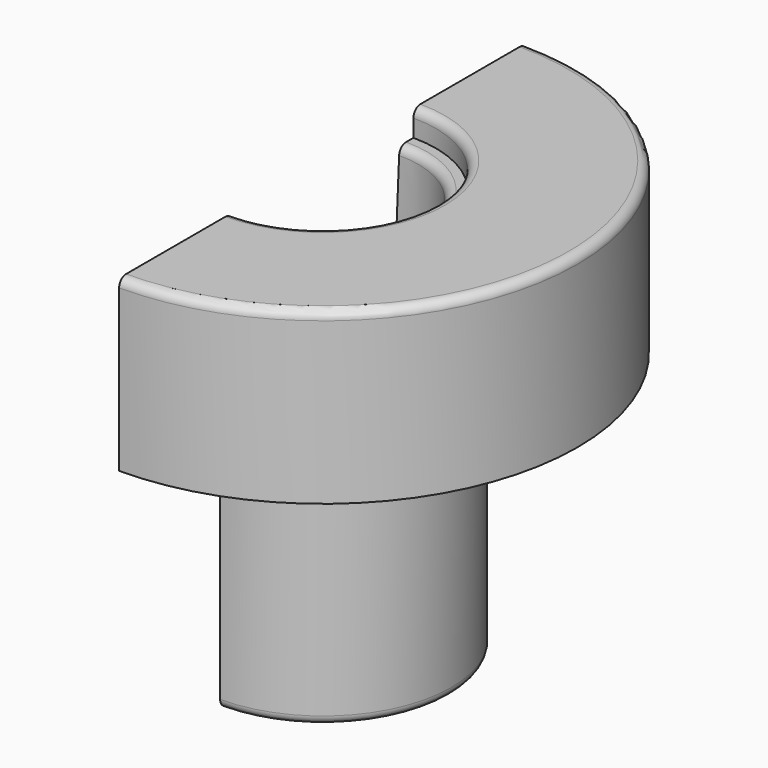
from build123d import *

# Parameters (mm, degrees)
F0_R         = 14.75
F1_DEPTH     = 30
F2_R         = 29.25
F3_DEPTH     = 19.5
F6_R         = 1
F8_W         = 73.76781106
F8_H         = 74.6486261487
F9_DEPTH     = 29.2510001
F10_T2_ANGLE = 183.7729101698
F11_R        = 1
F12_DEPTH    = 10


# Not quite as in the source:
# - a fillet or chamfer that OpenCascade refuses, or shapes differently, is made with other operations: its cross-section is extruded or revolved along the edge and cut away or added


with BuildPart() as f1:
    # F0 (on Top) → F1 (new body)
    with BuildSketch(Plane.XY):
        Circle(F0_R)
    extrude(amount=-F1_DEPTH)

    # F2 (on face) → F3 (join)
    with BuildSketch(Plane.XY):
        Circle(F2_R)
    extrude(amount=F3_DEPTH)

    # F4 (on Right) → F5 (revolve, cut)
    with BuildSketch(Plane.YZ):
        Polygon((13, 16.5), (13, 19.5), (0, 19.5), (0, -30), (10, -30), (10, -2.5), (11, 16.5), align=None)
    revolve(axis=Axis((0, 0, 5.2055120468), (0, 0, -1)), mode=Mode.SUBTRACT)

    # F6
    f6_edges = [f1.edges().sort_by_distance(p)[0] for p in [
        (-29.25, 0, 19.5),
        (0, -11, 16.5),
        (0, -13, 19.5),
        (0, -10, -30),
        (-14.75, 0, -30),
    ]]
    fillet(f6_edges, radius=F6_R)

    # F8 (on offset) → F9 (cut, through all)
    with BuildSketch(Plane.YZ):
        Rectangle(F8_W, F8_H)
    extrude(amount=-F9_DEPTH, mode=Mode.SUBTRACT)

    # F10: fillet of radius 5 on 1 edges, made by hand

    # F10_s1 → F10_t2 (revolve, cut)
    with BuildSketch(Plane(origin=(0, 0, 0), x_dir=(0, 0, 1), z_dir=(-0.999458026, -0.0329189041, 0))):
        with BuildLine():
            ThreePointArc((-2.6314879522, 10), (-2.5000454426, 10.0017280119), (-2.3686937866, 10.0069108533))
            Line((-2.3686937866, 10.0069108533), (-2.5, 10))
            Line((-2.5, 10), (-2.6314879522, 10))
        make_face()
    revolve(axis=Axis((0, 0, -2.5), (0, 0, -1)), revolution_arc=F10_T2_ANGLE, mode=Mode.SUBTRACT)

    # F11 (on face) → F12 (cut)
    with BuildSketch(Plane(origin=(0, 0, 0), x_dir=(0, -1, 0), z_dir=(-1, 0, 0))):
        with Locations((-21.587398374, 9.1951219512)):
            Circle(F11_R)
        with Locations((21.587398374, 9.1951219512)):
            Circle(F11_R)
    extrude(amount=-F12_DEPTH, mode=Mode.SUBTRACT)


solid = f1.part
